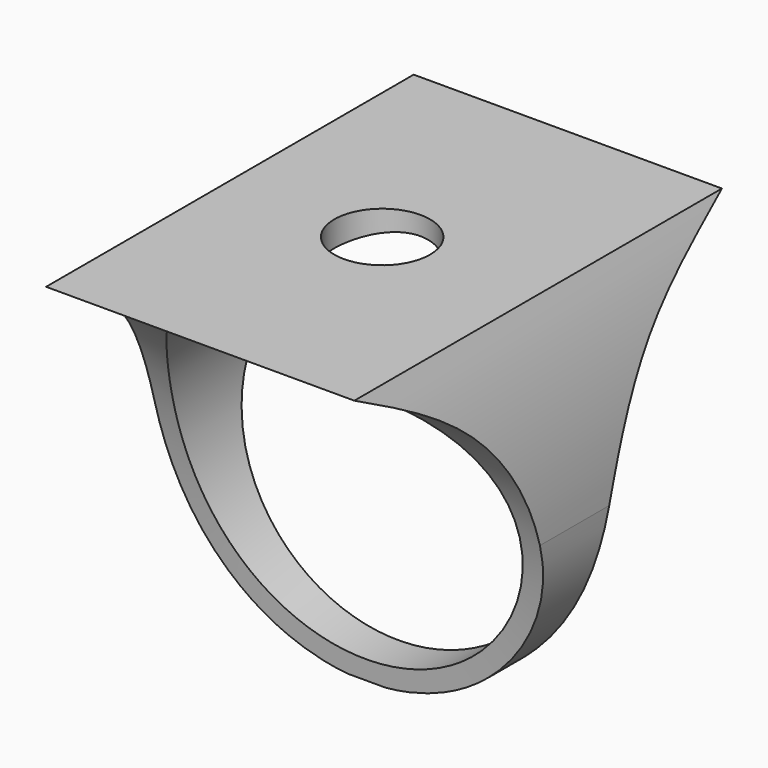
from build123d import *

# Parameters (mm, degrees)
F0_W     = 22
F0_H     = 20
F1_DEPTH = 12
F3_DEPTH = 25.4
F5_DEPTH = 12.7
F6_R     = 9
F7_DEPTH = 12.7
F8_R     = 2.5
F9_DEPTH = 5


with BuildPart() as f1:
    # F0 (on Front) → F1 (new body, symmetric)
    with BuildSketch(Plane.XZ):
        with Locations((0, -10)):
            Rectangle(F0_W, F0_H)
    extrude(amount=F1_DEPTH, both=True)

    # F2 (on face) → F3 (cut)
    with BuildSketch(Plane.YZ.offset(11)):
        with BuildLine():
            add(Edge.make_bspline(
                [(-1, -20), (-1.2459891412, -16.2571385999), (-1.6894774711, -9.5092173589), (-5.4667997235, -3.2161121648), (-9.8077344698, -1.0791911379), (-12, 0)],
                knots=[0, 0, 0, 0, 0.3813816119, 0.6875843918, 1, 1, 1, 1], degree=3))
            Line((-12, 0), (-12, -20))
            Line((-12, -20), (-1, -20))
        make_face()
        with BuildLine():
            Line((12, -20), (12, 0))
            add(Edge.make_bspline(
                [(1, -20), (1.2459891412, -16.2571385999), (1.6894774711, -9.5092173589), (5.4667997235, -3.2161121648), (9.8077344698, -1.0791911379), (12, 0)],
                knots=[0, 0, 0, 0, 0.3813816119, 0.6875843918, 1, 1, 1, 1], degree=3))
            Line((1, -20), (12, -20))
        make_face()
    extrude(amount=-F3_DEPTH, mode=Mode.SUBTRACT)

    # F4 (on Front) → F5 (cut, symmetric)
    with BuildSketch(Plane.XZ):
        with BuildLine():
            Line((11.243651621, 0), (8.1397629196, 0.0138028498))
            ThreePointArc((8.1397629196, 0.0138028498), (9.568173485, -4.902813197), (10.05, -10))
            ThreePointArc((10.05, -10), (7.1064231509, -17.1064231509), (0, -20.05))
            Line((0, -20.05), (11.243651621, -20.0490429997))
            Line((11.243651621, -20.0490429997), (11.243651621, 0))
        make_face()
        with BuildLine():
            ThreePointArc((-10.05, -10), (-9.5188754702, -4.8835783868), (-7.9481515297, 0.0146549369))
            Line((-7.9481515297, 0.0146549369), (-10.05, 0.0053081137))
            Line((-10.05, 0.0053081137), (-11.243651621, 0))
            Line((-11.243651621, 0), (-11.243651621, -20.0490429997))
            Line((-11.243651621, -20.0490429997), (0, -20.05))
            ThreePointArc((0, -20.05), (-7.1064231509, -17.1064231509), (-10.05, -10))
        make_face()
    extrude(amount=F5_DEPTH, both=True, mode=Mode.SUBTRACT)

    # F6 (on Front) → F7 (cut, symmetric)
    with BuildSketch(Plane.XZ):
        with Locations((0, -9.9779)):
            Circle(F6_R)
    extrude(amount=F7_DEPTH, both=True, mode=Mode.SUBTRACT)

    # F8 (on face) → F9 (cut)
    with BuildSketch(Plane.XY):
        Circle(F8_R)
    extrude(amount=-F9_DEPTH, mode=Mode.SUBTRACT)


solid = f1.part
